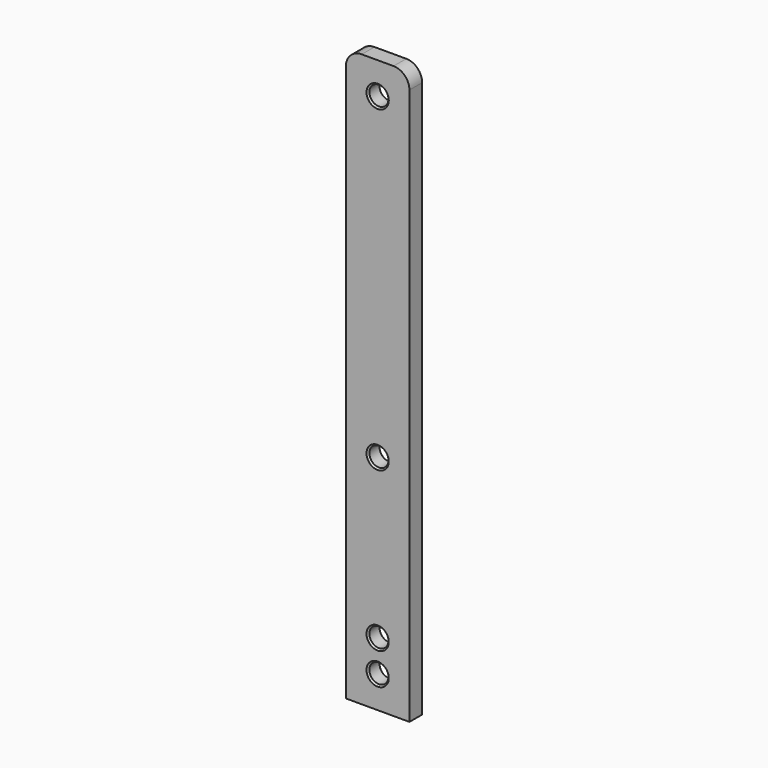
from build123d import *

# Parameters (mm, degrees)
F0_W     = 20
F0_H     = 180
F1_DEPTH = 5
F2_R     = 3
F3_DEPTH = 5.001
F5_D     = 6
F7_D     = 6
F8_SIZE  = 0.5
F9_R     = 5


with BuildPart() as f1:
    # F0 (on Front) → F1 (new body)
    with BuildSketch(Plane.XZ):
        with Locations((10, 90)):
            Rectangle(F0_W, F0_H)
    extrude(amount=F1_DEPTH)

    # F2 (on face) → F3 (cut, through all)
    with BuildSketch(Plane.XZ.offset(5)):
        with Locations((10, 170)):
            Circle(F2_R)
    extrude(amount=-F3_DEPTH, mode=Mode.SUBTRACT)

    # F5 (through all)
    with Locations(Plane.XZ.offset(5)):
        with Locations((10, 70)):
            Hole(F5_D / 2)

    # F7 (through all)
    with Locations(Plane.XZ.offset(5)):
        with Locations((10, 10), (10, 20)):
            Hole(F7_D / 2)

    # F8
    f8_edges = [f1.edges().sort_by_distance(p)[0] for p in [
        (7, -5, 170),
        (7, 0, 170),
        (7, 0, 10),
        (7, 0, 20),
        (7, 0, 70),
        (7, -5, 10),
        (7, -5, 20),
        (7, -5, 70),
    ]]
    chamfer(f8_edges, length=F8_SIZE)

    # F9
    f9_edges = [f1.edges().sort_by_distance(p)[0] for p in [
        (20, -2.5, 180),
        (0, -2.5, 180),
    ]]
    fillet(f9_edges, radius=F9_R)


solid = f1.part
